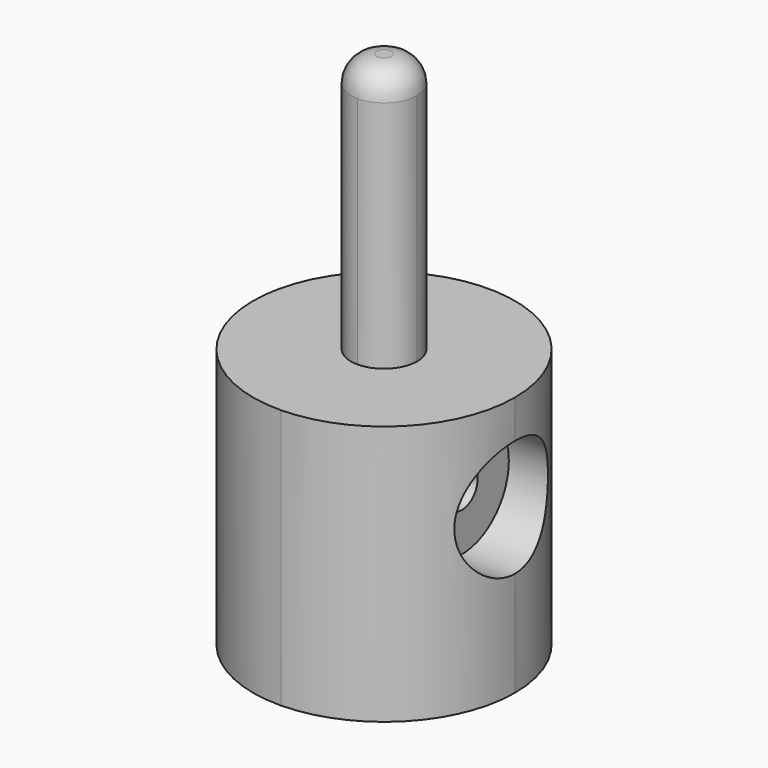
from build123d import *

# Parameters (mm, degrees)
F1_DEPTH  = 10
F2_DEPTH  = 10
F4_R      = 1.2735627731
F5_DEPTH  = 8
F6_R      = 0.75
F7_DEPTH  = 12.5
F9_R      = 2.25
F9_R_2    = 0.75
F10_DEPTH = 2
F12_R     = 2.25
F12_R_2   = 0.75
F13_DEPTH = 2


# Not quite as in the source:
# - a fillet or chamfer that OpenCascade refuses, or shapes differently, is made with other operations: its cross-section is extruded or revolved along the edge and cut away or added
# - a feature names something its author has since deleted; it is built from what else it names


with BuildPart() as f1:
    # F0 (on Top) → F1 (new body)
    with BuildSketch(Plane.XY):
        with BuildLine():
            Line((0, 0), (1.2735627731, 0))
            ThreePointArc((1.2735627731, 0), (0.9005448731, 0.9005448731), (0, 1.2735627731))
            Line((0, 1.2735627731), (0, 0))
        make_face()
        with BuildLine():
            Line((0, 0), (0, 1.2735627731))
            ThreePointArc((0, 1.2735627731), (-0.9005448731, 0.9005448731), (-1.2735627731, 0))
            Line((-1.2735627731, 0), (0, 0))
        make_face()
        with BuildLine():
            ThreePointArc((-1.2735627731, 0), (-0.9005448731, -0.9005448731), (0, -1.2735627731))
            Line((0, -1.2735627731), (0, 0))
            Line((0, 0), (-1.2735627731, 0))
        make_face()
        with BuildLine():
            ThreePointArc((0, -1.2735627731), (0.9005448731, -0.9005448731), (1.2735627731, 0))
            Line((1.2735627731, 0), (0, 0))
            Line((0, 0), (0, -1.2735627731))
        make_face()
    extrude(amount=F1_DEPTH)

    # F0 (on Top) → F2 (join)
    with BuildSketch(Plane.XY):
        with BuildLine():
            ThreePointArc((0.0602184818, -5.0337774218), (3.5808999931, -3.5383183346), (5.0341376022, 0))
            ThreePointArc((5.0341376022, 0), (-0.0301919188, 5.0340470643), (-5.033775454, -0.0603827516))
            ThreePointArc((-5.033775454, -0.0603827516), (-3.5167784797, -3.6020564297), (0.0602184818, -5.0337774218))
        make_face()
        with BuildLine():
            ThreePointArc((0, 1.2735627731), (0.9005448731, 0.9005448731), (1.2735627731, 0))
            ThreePointArc((1.2735627731, 0), (0.9005448731, -0.9005448731), (0, -1.2735627731))
            ThreePointArc((0, -1.2735627731), (-0.9005448731, -0.9005448731), (-1.2735627731, 0))
            ThreePointArc((-1.2735627731, 0), (-0.9005448731, 0.9005448731), (0, 1.2735627731))
        make_face(mode=Mode.SUBTRACT)
        with BuildLine():
            Line((0, 0), (1.2735627731, 0))
            ThreePointArc((1.2735627731, 0), (0.9005448731, 0.9005448731), (0, 1.2735627731))
            Line((0, 1.2735627731), (0, 0))
        make_face()
        with BuildLine():
            Line((0, 0), (0, 1.2735627731))
            ThreePointArc((0, 1.2735627731), (-0.9005448731, 0.9005448731), (-1.2735627731, 0))
            Line((-1.2735627731, 0), (0, 0))
        make_face()
        with BuildLine():
            ThreePointArc((-1.2735627731, 0), (-0.9005448731, -0.9005448731), (0, -1.2735627731))
            Line((0, -1.2735627731), (0, 0))
            Line((0, 0), (-1.2735627731, 0))
        make_face()
        with BuildLine():
            ThreePointArc((0, -1.2735627731), (0.9005448731, -0.9005448731), (1.2735627731, 0))
            Line((1.2735627731, 0), (0, 0))
            Line((0, 0), (0, -1.2735627731))
        make_face()
    extrude(amount=-F2_DEPTH)

    # F3: fillet of radius 1 on 1 edges, made by hand

    # F3_s1 → F3_t2 (revolve, cut)
    with BuildSketch(Plane.YZ):
        with BuildLine():
            ThreePointArc((-1.2735627731, 9), (-0.9806695543, 9.7071067812), (-0.2735627731, 10))
            Line((-0.2735627731, 10), (-1.2735627731, 10))
            Line((-1.2735627731, 10), (-1.2735627731, 9))
        make_face()
    revolve(axis=Axis((0, 0, 10), (0, 0, 1)), mode=Mode.SUBTRACT)

    # F4 (on face) → F5 (cut)
    with BuildSketch(Plane(origin=(0, 0, -10), x_dir=(1, 0, 0), z_dir=(0, 0, -1))):
        Circle(F4_R)
    extrude(amount=-F5_DEPTH, mode=Mode.SUBTRACT)

    # F6 (on Right) → F7 (cut, symmetric)
    with BuildSketch(Plane.YZ):
        with Locations((0, -3.7172080483)):
            Circle(F6_R)
    extrude(amount=F7_DEPTH, both=True, mode=Mode.SUBTRACT)

    # F9 (on offset) → F10 (cut, symmetric)
    with BuildSketch(Plane.YZ.offset(5)):
        with Locations((0, -3.7172080483)):
            Circle(F9_R)
        with Locations((0, -3.7172080483)):
            Circle(F9_R_2, mode=Mode.SUBTRACT)
    extrude(amount=F10_DEPTH, both=True, mode=Mode.SUBTRACT)

    # F12 (on offset) → F13 (cut, symmetric)
    with BuildSketch(Plane.YZ.offset(-5)):
        with Locations((0, -3.7172080483)):
            Circle(F12_R)
        with Locations((0, -3.7172080483)):
            Circle(F12_R_2, mode=Mode.SUBTRACT)
    extrude(amount=F13_DEPTH, both=True, mode=Mode.SUBTRACT)


solid = f1.part
